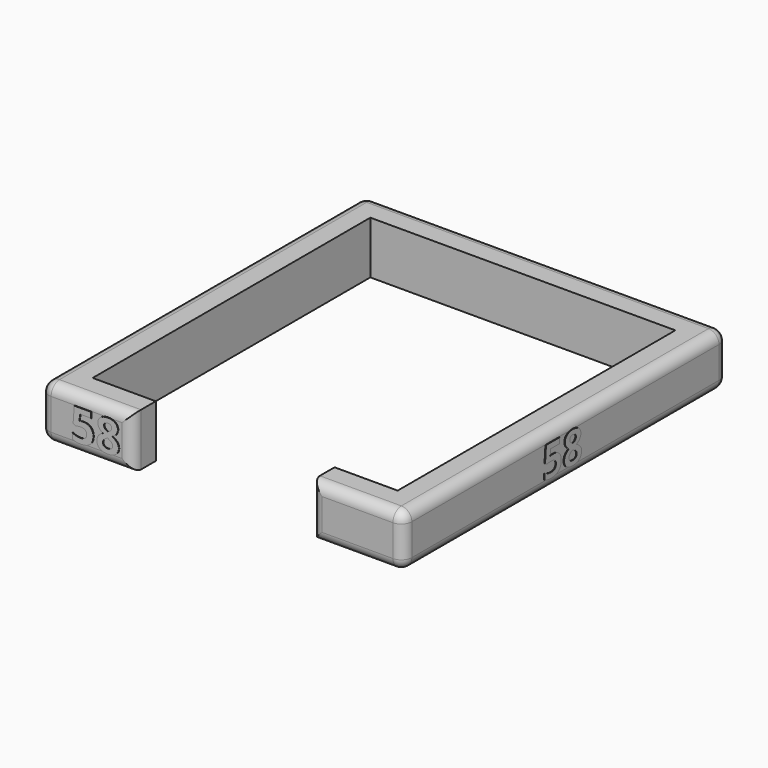
from build123d import *

# Parameters (mm, degrees)
F1_DEPTH     = 127
F2_T1_DEPTH  = 927.1
F2_T3_DEPTH  = 260.35
F2_T5_DEPTH  = 825.5
F2_T7_DEPTH  = 1016
F2_T9_DEPTH  = 349.25
F2_T11_DEPTH = 254
F2_T13_DEPTH = 76.2
F2_S17_W     = 25.908
F2_S17_H     = 25.908
F2_T18_DEPTH = 25.908
F2_S23_W     = 25.908
F2_S23_H     = 25.908
F2_T24_DEPTH = 25.908
F2_S29_W     = 25.908
F2_S29_H     = 25.908
F2_T30_DEPTH = 25.908
F2_S35_W     = 25.908
F2_S35_H     = 25.908
F2_T36_DEPTH = 25.908
F2_S41_W     = 25.908
F2_S41_H     = 25.908
F2_T42_DEPTH = 25.908
F2_S47_W     = 25.908
F2_S47_H     = 25.908
F2_T48_DEPTH = 25.908
F3_TEXT_SIZE = 105.8333333333
F4_DEPTH     = 1.27
F7_T1_DEPTH  = 76.2
F7_S5_W      = 25.4
F7_S5_H      = 25.4
F7_T6_DEPTH  = 25.4
F7_S11_W     = 25.4
F7_S11_H     = 25.4
F7_T12_DEPTH = 25.4
F8_TEXT_SIZE = 105.8333333333
F9_DEPTH     = 1.27
F5_TEXT_SIZE = 105.8333333333
F10_DEPTH    = 1.27
F6_TEXT_SIZE = 105.8333333333
F11_DEPTH    = 1.27


# Not quite as in the source:
# - a fillet or chamfer that OpenCascade refuses, or shapes differently, is made with other operations: its cross-section is extruded or revolved along the edge and cut away or added
# - Text() gives the source's letters only with a copy of the font that has no kerning and outlines rounded to 1/6400 em; it was checked with that copy


with BuildPart() as f1:
    # F0 (on Top) → F1 (new body)
    with BuildSketch(Plane.XY):
        Polygon((-368.3, 419.1), (368.3, 419.1), (368.3, -419.1), (215.9, -419.1), (215.9, -488.95), (438.15, -488.95), (438.15, 488.95), (-438.15, 488.95), (-438.15, -488.95), (-215.9, -488.95), (-215.9, -419.1), (-368.3, -419.1), align=None)
    extrude(amount=F1_DEPTH)

    # F2: fillet of radius 25.4 on 15 edges, made by hand

    # F2_s2 → F2_t1 (cut)
    with BuildSketch(Plane.XZ.offset(-463.55)):
        with BuildLine():
            ThreePointArc((438.15, 101.6), (430.7105122421, 119.5605122421), (412.75, 127))
            Line((412.75, 127), (438.15, 127))
            Line((438.15, 127), (438.15, 101.6))
        make_face()
        with BuildLine():
            ThreePointArc((438.15, 25.4), (430.7105122421, 7.4394877579), (412.75, 0))
            Line((412.75, 0), (438.15, 0))
            Line((438.15, 0), (438.15, 25.4))
        make_face()
    extrude(amount=F2_T1_DEPTH, mode=Mode.SUBTRACT)

    # F2_s4 → F2_t3 (cut)
    with BuildSketch(Plane.YZ.offset(152.4)):
        with BuildLine():
            ThreePointArc((-488.95, 101.6), (-481.5105122421, 119.5605122421), (-463.55, 127))
            Line((-463.55, 127), (-488.95, 127))
            Line((-488.95, 127), (-488.95, 101.6))
        make_face()
        with BuildLine():
            ThreePointArc((-488.95, 25.4), (-481.5105122421, 7.4394877579), (-463.55, 0))
            Line((-463.55, 0), (-488.95, 0))
            Line((-488.95, 0), (-488.95, 25.4))
        make_face()
    extrude(amount=F2_T3_DEPTH, mode=Mode.SUBTRACT)

    # F2_s6 → F2_t5 (cut)
    with BuildSketch(Plane.YZ.offset(-412.75)):
        with BuildLine():
            ThreePointArc((488.95, 101.6), (481.5105122421, 119.5605122421), (463.55, 127))
            Line((463.55, 127), (488.95, 127))
            Line((488.95, 127), (488.95, 101.6))
        make_face()
        with BuildLine():
            ThreePointArc((488.95, 25.4), (481.5105122421, 7.4394877579), (463.55, 0))
            Line((463.55, 0), (488.95, 0))
            Line((488.95, 0), (488.95, 25.4))
        make_face()
    extrude(amount=F2_T5_DEPTH, mode=Mode.SUBTRACT)

    # F2_s8 → F2_t7 (cut)
    with BuildSketch(Plane.XZ.offset(-463.55)):
        with BuildLine():
            ThreePointArc((-438.15, 101.6), (-430.7105122421, 119.5605122421), (-412.75, 127))
            Line((-412.75, 127), (-438.15, 127))
            Line((-438.15, 127), (-438.15, 101.6))
        make_face()
        with BuildLine():
            ThreePointArc((-438.15, 25.4), (-430.7105122421, 7.4394877579), (-412.75, 0))
            Line((-412.75, 0), (-438.15, 0))
            Line((-438.15, 0), (-438.15, 25.4))
        make_face()
    extrude(amount=F2_T7_DEPTH, mode=Mode.SUBTRACT)

    # F2_s10 → F2_t9 (cut)
    with BuildSketch(Plane.YZ.offset(-501.65)):
        with BuildLine():
            ThreePointArc((-488.95, 101.6), (-481.5105122421, 119.5605122421), (-463.55, 127))
            Line((-463.55, 127), (-488.95, 127))
            Line((-488.95, 127), (-488.95, 101.6))
        make_face()
        with BuildLine():
            ThreePointArc((-488.95, 25.4), (-481.5105122421, 7.4394877579), (-463.55, 0))
            Line((-463.55, 0), (-488.95, 0))
            Line((-488.95, 0), (-488.95, 25.4))
        make_face()
    extrude(amount=F2_T9_DEPTH, mode=Mode.SUBTRACT)

    # F2_s12 → F2_t11 (cut)
    with BuildSketch(Plane.XY.offset(-63.5)):
        with BuildLine():
            ThreePointArc((-241.3, -488.95), (-223.3394877579, -481.5105122421), (-215.9, -463.55))
            Line((-215.9, -463.55), (-215.9, -488.95))
            Line((-215.9, -488.95), (-241.3, -488.95))
        make_face()
        with BuildLine():
            ThreePointArc((215.9, -463.55), (223.3394877579, -481.5105122421), (241.3, -488.95))
            Line((241.3, -488.95), (215.9, -488.95))
            Line((215.9, -488.95), (215.9, -463.55))
        make_face()
    extrude(amount=F2_T11_DEPTH, mode=Mode.SUBTRACT)

    # F2_s14 → F2_t13 (cut)
    with BuildSketch(Plane.XY.offset(25.4)):
        with BuildLine():
            ThreePointArc((-412.75, 488.95), (-430.7105122421, 481.5105122421), (-438.15, 463.55))
            Line((-438.15, 463.55), (-438.15, 488.95))
            Line((-438.15, 488.95), (-412.75, 488.95))
        make_face()
        with BuildLine():
            ThreePointArc((438.15, 463.55), (430.7105122421, 481.5105122421), (412.75, 488.95))
            Line((412.75, 488.95), (438.15, 488.95))
            Line((438.15, 488.95), (438.15, 463.55))
        make_face()
        with BuildLine():
            ThreePointArc((412.75, -488.95), (430.7105122421, -481.5105122421), (438.15, -463.55))
            Line((438.15, -463.55), (438.15, -488.95))
            Line((438.15, -488.95), (412.75, -488.95))
        make_face()
    extrude(amount=F2_T13_DEPTH, mode=Mode.SUBTRACT)


with BuildPart() as f2_tool16:
    # F2_s17 → F2_t18 (new body)
    with BuildSketch(Plane.XY.offset(101.6)):
        with Locations((425.704, -476.504)):
            Rectangle(F2_S17_W, F2_S17_H)
    extrude(amount=F2_T18_DEPTH)

    # F2_s19 → F2_t20 (revolve, cut)
    with BuildSketch(Plane(origin=(412.75, -463.55, 101.6), x_dir=(-0.7071067812, 0.7071067812, 0), z_dir=(0.7071067812, 0.7071067812, 0))):
        with BuildLine():
            ThreePointArc((0, -25.4), (25.4, 0), (0, 25.4))
            Line((0, 25.4), (0, -25.4))
        make_face()
    revolve(axis=Axis((412.75, -463.55, 101.6), (0, 0, 1)), mode=Mode.SUBTRACT)


with BuildPart() as f1_1:
    add(f1.part)

    # F2_t15: cut F2_tool16
    add(f2_tool16.part, mode=Mode.SUBTRACT)


with BuildPart() as f2_tool22:
    # F2_s23 → F2_t24 (new body)
    with BuildSketch(Plane.XY.offset(101.6)):
        with Locations((425.704, 476.504)):
            Rectangle(F2_S23_W, F2_S23_H)
    extrude(amount=F2_T24_DEPTH)

    # F2_s25 → F2_t26 (revolve, cut)
    with BuildSketch(Plane(origin=(412.75, 463.55, 101.6), x_dir=(-0.7071067812, -0.7071067812, 0), z_dir=(-0.7071067812, 0.7071067812, 0))):
        with BuildLine():
            ThreePointArc((0, -25.4), (25.4, 0), (0, 25.4))
            Line((0, 25.4), (0, -25.4))
        make_face()
    revolve(axis=Axis((412.75, 463.55, 101.6), (0, 0, 1)), mode=Mode.SUBTRACT)


with BuildPart() as f1_2:
    add(f1_1.part)

    # F2_t21: cut F2_tool22
    add(f2_tool22.part, mode=Mode.SUBTRACT)


with BuildPart() as f2_tool28:
    # F2_s29 → F2_t30 (new body)
    with BuildSketch(Plane.XY.offset(101.6)):
        with Locations((-425.704, 476.504)):
            Rectangle(F2_S29_W, F2_S29_H)
    extrude(amount=F2_T30_DEPTH)

    # F2_s31 → F2_t32 (revolve, cut)
    with BuildSketch(Plane(origin=(-412.75, 463.55, 101.6), x_dir=(0.7071067812, -0.7071067812, 0), z_dir=(-0.7071067812, -0.7071067812, 0))):
        with BuildLine():
            ThreePointArc((0, -25.4), (25.4, 0), (0, 25.4))
            Line((0, 25.4), (0, -25.4))
        make_face()
    revolve(axis=Axis((-412.75, 463.55, 101.6), (0, 0, 1)), mode=Mode.SUBTRACT)


with BuildPart() as f1_3:
    add(f1_2.part)

    # F2_t27: cut F2_tool28
    add(f2_tool28.part, mode=Mode.SUBTRACT)


with BuildPart() as f2_tool34:
    # F2_s35 → F2_t36 (new body)
    with BuildSketch(Plane.XY.offset(25.4)):
        with Locations((-425.704, 476.504)):
            Rectangle(F2_S35_W, F2_S35_H)
    extrude(amount=-F2_T36_DEPTH)

    # F2_s37 → F2_t38 (revolve, cut)
    with BuildSketch(Plane(origin=(-412.75, 463.55, 25.4), x_dir=(0.7071067812, -0.7071067812, 0), z_dir=(0.7071067812, 0.7071067812, 0))):
        with BuildLine():
            ThreePointArc((0, -25.4), (25.4, 0), (0, 25.4))
            Line((0, 25.4), (0, -25.4))
        make_face()
    revolve(axis=Axis((-412.75, 463.55, 25.4), (0, 0, -1)), mode=Mode.SUBTRACT)


with BuildPart() as f1_4:
    add(f1_3.part)

    # F2_t33: cut F2_tool34
    add(f2_tool34.part, mode=Mode.SUBTRACT)


with BuildPart() as f2_tool40:
    # F2_s41 → F2_t42 (new body)
    with BuildSketch(Plane.XY.offset(25.4)):
        with Locations((425.704, 476.504)):
            Rectangle(F2_S41_W, F2_S41_H)
    extrude(amount=-F2_T42_DEPTH)

    # F2_s43 → F2_t44 (revolve, cut)
    with BuildSketch(Plane(origin=(412.75, 463.55, 25.4), x_dir=(-0.7071067812, -0.7071067812, 0), z_dir=(0.7071067812, -0.7071067812, 0))):
        with BuildLine():
            ThreePointArc((0, -25.4), (25.4, 0), (0, 25.4))
            Line((0, 25.4), (0, -25.4))
        make_face()
    revolve(axis=Axis((412.75, 463.55, 25.4), (0, 0, -1)), mode=Mode.SUBTRACT)


with BuildPart() as f1_5:
    add(f1_4.part)

    # F2_t39: cut F2_tool40
    add(f2_tool40.part, mode=Mode.SUBTRACT)


with BuildPart() as f2_tool46:
    # F2_s47 → F2_t48 (new body)
    with BuildSketch(Plane.XZ.offset(463.55)):
        with Locations((425.704, 12.446)):
            Rectangle(F2_S47_W, F2_S47_H)
    extrude(amount=F2_T48_DEPTH)

    # F2_s49 → F2_t50 (revolve, cut)
    with BuildSketch(Plane(origin=(412.75, -463.55, 25.4), x_dir=(-0.7071067812, 0, 0.7071067812), z_dir=(0.7071067812, 0, 0.7071067812))):
        with BuildLine():
            ThreePointArc((0, -25.4), (25.4, 0), (0, 25.4))
            Line((0, 25.4), (0, -25.4))
        make_face()
    revolve(axis=Axis((412.75, -463.55, 25.4), (0, -1, 0)), mode=Mode.SUBTRACT)


with BuildPart() as f1_6:
    add(f1_5.part)

    # F2_t45: cut F2_tool46
    add(f2_tool46.part, mode=Mode.SUBTRACT)

    # F7: fillet of radius 25.4 on 1 edges, made by hand

    # F7_s2 → F7_t1 (cut)
    with BuildSketch(Plane.XY.offset(25.4)):
        with BuildLine():
            ThreePointArc((-438.15, -463.55), (-430.7105122421, -481.5105122421), (-412.75, -488.95))
            Line((-412.75, -488.95), (-438.15, -488.95))
            Line((-438.15, -488.95), (-438.15, -463.55))
        make_face()
    extrude(amount=F7_T1_DEPTH, mode=Mode.SUBTRACT)


with BuildPart() as f4:
    # F3 (on face) → F4 (new body)
    with BuildSketch(Plane.YZ.offset(438.15)):
        with Locations((-69.85, 25.4)):
            Text('58', F3_TEXT_SIZE, font='Open Sans', font_style=FontStyle.BOLD, text_align=(TextAlign.LEFT, TextAlign.BOTTOM))
    extrude(amount=F4_DEPTH)


with BuildPart() as f7_tool4:
    # F7_s5 → F7_t6 (new body)
    with BuildSketch(Plane.YZ.offset(-412.75)):
        with Locations((-476.25, 12.7)):
            Rectangle(F7_S5_W, F7_S5_H)
    extrude(amount=-F7_T6_DEPTH)

    # F7_s7 → F7_t8 (revolve, cut)
    with BuildSketch(Plane(origin=(-412.75, -463.55, 25.4), x_dir=(0, 0.7071067812, 0.7071067812), z_dir=(0, -0.7071067812, 0.7071067812))):
        with BuildLine():
            ThreePointArc((0, -25.4), (25.4, 0), (0, 25.4))
            Line((0, 25.4), (0, -25.4))
        make_face()
    revolve(axis=Axis((-412.75, -463.55, 25.4), (-1, 0, 0)), mode=Mode.SUBTRACT)


with BuildPart() as f1_7:
    add(f1_6.part)

    # F7_t3: cut F7_tool4
    add(f7_tool4.part, mode=Mode.SUBTRACT)


with BuildPart() as f7_tool10:
    # F7_s11 → F7_t12 (new body)
    with BuildSketch(Plane.YZ.offset(-412.75)):
        with Locations((-476.25, 114.3)):
            Rectangle(F7_S11_W, F7_S11_H)
    extrude(amount=-F7_T12_DEPTH)

    # F7_s13 → F7_t14 (revolve, cut)
    with BuildSketch(Plane(origin=(-412.75, -463.55, 101.6), x_dir=(0, 0.7071067812, -0.7071067812), z_dir=(0, 0.7071067812, 0.7071067812))):
        with BuildLine():
            ThreePointArc((0, -25.4), (25.4, 0), (0, 25.4))
            Line((0, 25.4), (0, -25.4))
        make_face()
    revolve(axis=Axis((-412.75, -463.55, 101.6), (-1, 0, 0)), mode=Mode.SUBTRACT)


with BuildPart() as f1_8:
    add(f1_7.part)

    # F7_t9: cut F7_tool10
    add(f7_tool10.part, mode=Mode.SUBTRACT)


with BuildPart() as f9:
    # F8 (on face) → F9 (new body)
    with BuildSketch(Plane.XZ.offset(488.95)):
        with Locations((-365.3069010417, 25.4)):
            Text('58', F8_TEXT_SIZE, font='Open Sans', font_style=FontStyle.BOLD, text_align=(TextAlign.LEFT, TextAlign.BOTTOM))
    extrude(amount=F9_DEPTH)


with BuildPart() as f10:
    # F5 (on face) → F10 (new body)
    with BuildSketch(Plane(origin=(-438.15, 0, 0), x_dir=(0, -1, 0), z_dir=(-1, 0, 0))):
        with Locations((-28.7569010417, 25.4)):
            Text('58', F5_TEXT_SIZE, font='Open Sans', font_style=FontStyle.BOLD, text_align=(TextAlign.LEFT, TextAlign.BOTTOM))
    extrude(amount=F10_DEPTH)


with BuildPart() as f11:
    # F6 (on face) → F11 (new body)
    with BuildSketch(Plane(origin=(0, 488.95, 0), x_dir=(-1, 0, 0), z_dir=(0, 1, 0))):
        with Locations((-66.8569010417, 25.4)):
            Text('58', F6_TEXT_SIZE, font='Open Sans', font_style=FontStyle.BOLD, text_align=(TextAlign.LEFT, TextAlign.BOTTOM))
    extrude(amount=F11_DEPTH)


solid = Compound([f4.part, f1_8.part, f9.part, f10.part, f11.part])
